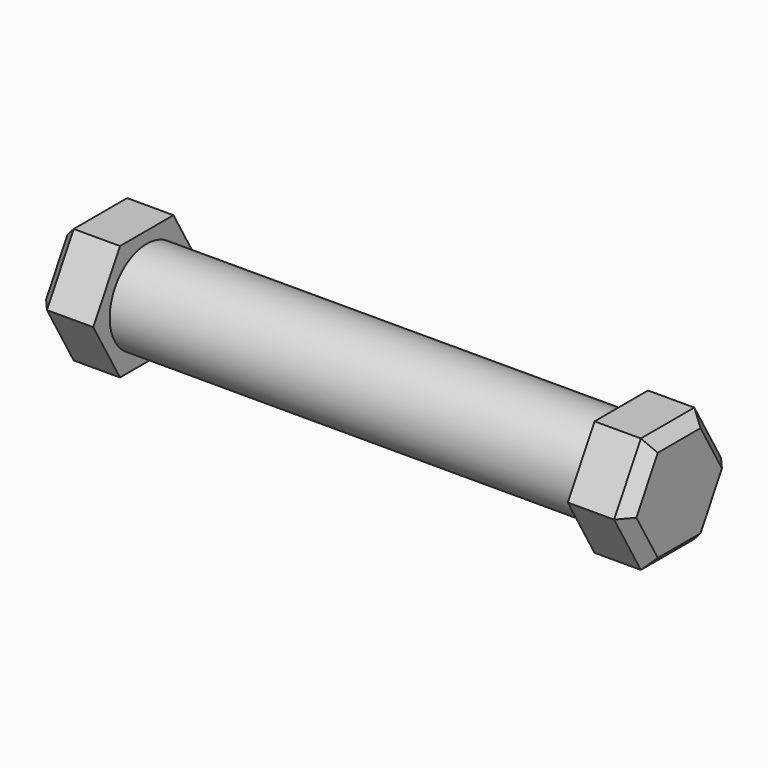
from build123d import *

# Parameters (mm, degrees)
F0_R     = 4
F1_DEPTH = 20.5
F3_DEPTH = 5
F4_SIZE  = 1


# Not quite as in the source:
# - a pattern or mirror of a feature is missing from the dataset's text; its kind, count and spacing are read off the source's solid


with BuildPart() as f1:
    # F0 (on Right) → F1 (new body, symmetric)
    with BuildSketch(Plane.YZ):
        Circle(F0_R)
    extrude(amount=F1_DEPTH, both=True)

    # F2 (on face) → F3 (join)
    with BuildSketch(Plane.YZ.offset(20.5)):
        Polygon((2.8867513459, 5), (-2.8867513459, 5), (-5.7735026919, 0), (-2.8867513459, -5), (2.8867513459, -5), (5.7735026919, 0), align=None)
    f3 = extrude(amount=F3_DEPTH)

    # F3_copies: F3 across plane
    add(f3.mirror(Plane(origin=(0, 0, 0), x_dir=(0, 0, -1), z_dir=(-1, 0, 0))))

    # F4
    f4_edges = [f1.edges().sort_by_distance(p)[0] for p in [
        (25.5, 4.330127, 2.5),
        (25.5, 0, 5),
        (25.5, -4.330127, 2.5),
        (25.5, -4.330127, -2.5),
        (25.5, 0, -5),
        (25.5, 4.330127, -2.5),
        (-25.5, 4.330127, 2.5),
        (-25.5, 4.330127, -2.5),
        (-25.5, 0, 5),
        (-25.5, -4.330127, 2.5),
        (-25.5, -4.330127, -2.5),
        (-25.5, 0, -5),
    ]]
    chamfer(f4_edges, length=F4_SIZE)


solid = f1.part
